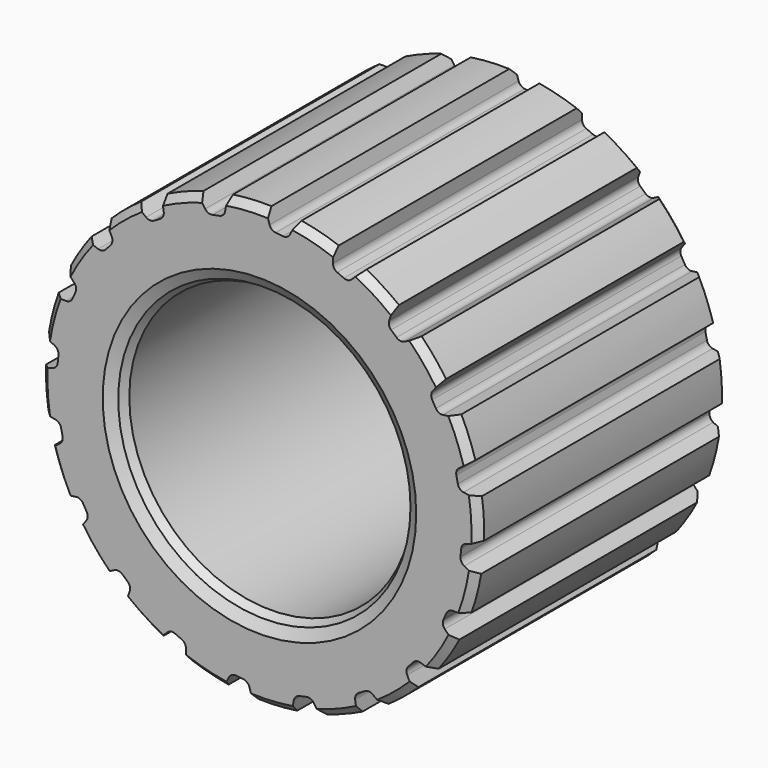
from build123d import *

# Parameters (mm, degrees)
F0_R            = 15.485
F0_R_2          = 10
F1_DEPTH        = 11
F2_SIZE2        = 0.5773502692
F2_SIZE         = 1
F3_SIZE2        = 0.5
F3_SIZE         = 0.5
F5_DEPTH        = 12.5
F5_COPIES_COUNT = 20
F6_SIZE2        = 0.5
F6_SIZE         = 0.5


# Not quite as in the source:
# - a pattern or mirror of a feature is missing from the dataset's text; its kind, count and spacing are read off the source's solid


with BuildPart() as f1:
    # F0 (on Front) → F1 (new body, symmetric)
    with BuildSketch(Plane.XZ):
        Circle(F0_R)
        Circle(F0_R_2, mode=Mode.SUBTRACT)
    extrude(amount=F1_DEPTH, both=True)

    # F2
    f2_edges = [f1.edges().sort_by_distance(p)[0] for p in [
        (-10, -11, 0),
        (-10, 11, 0),
    ]]
    f2_side = f1.faces().sort_by_distance((-10, 0, 0))[0]
    chamfer(f2_edges, length=F2_SIZE, length2=F2_SIZE2, reference=f2_side)

    # F3
    f3_edges = [f1.edges().sort_by_distance(p)[0] for p in [
        (-10.57735, -11, 0),
        (-10.57735, 11, 0),
    ]]
    chamfer(f3_edges, length=F3_SIZE, length2=F3_SIZE2)

    # F4 (on Front) → F5 (cut, symmetric)
    with BuildSketch(Plane.XZ):
        with BuildLine():
            Line((-2.4258394789, 14.4213544606), (-2.2677279827, 15.3180493143))
            ThreePointArc((-2.2677279827, 15.3180493143), (-3.319655777, 15.1249829925), (-4.3557481049, 14.8597672743))
            Line((-4.3557481049, 14.8597672743), (-3.8334908043, 14.1139065515))
            ThreePointArc((-3.8334908043, 14.1139065515), (-3.6071653955, 13.9354859857), (-3.3199589368, 13.9116209693))
            Line((-3.3199589368, 13.9116209693), (-2.81428751, 14.0191047491))
            ThreePointArc((-2.81428751, 14.0191047491), (-2.5585734552, 14.1608493642), (-2.4258394789, 14.4213544606))
        make_face()
    f5 = extrude(amount=F5_DEPTH, both=True, mode=Mode.SUBTRACT)

    # F5_copies: F5 ×20 about axis
    f5_copies_axis = Axis((0, 0, 0), (0, 1, 0))
    for i in range(1, F5_COPIES_COUNT):
        add(f5.rotate(f5_copies_axis, i * 360 / F5_COPIES_COUNT), mode=Mode.SUBTRACT)

    # F6
    f6_edges = [f1.edges().sort_by_distance(p)[0] for p in [
        (-15.458078, 11, -0.912717),
        (-15.458078, -11, -0.912717),
        (-0.912717, -11, 15.458078),
        (3.908764, -11, 14.983551),
        (8.347627, -11, 13.042329),
        (11.969366, -11, 9.824434),
        (14.419461, -11, 5.644854),
        (15.458078, -11, 0.912717),
        (14.983551, -11, -3.908764),
        (13.042329, -11, -8.347627),
        (9.824434, -11, -11.969366),
        (5.644854, -11, -14.419461),
        (0.912717, -11, -15.458078),
        (-3.908764, -11, -14.983551),
        (-8.347627, -11, -13.042329),
        (-11.969366, -11, -9.824434),
        (-14.419461, -11, -5.644854),
        (-14.983551, -11, 3.908764),
        (-13.042329, -11, 8.347627),
        (-9.824434, -11, 11.969366),
        (-5.644854, -11, 14.419461),
        (-0.912717, 11, 15.458078),
        (3.908764, 11, 14.983551),
        (8.347627, 11, 13.042329),
        (11.969366, 11, 9.824434),
        (14.419461, 11, 5.644854),
        (15.458078, 11, 0.912717),
        (14.983551, 11, -3.908764),
        (13.042329, 11, -8.347627),
        (9.824434, 11, -11.969366),
        (5.644854, 11, -14.419461),
        (0.912717, 11, -15.458078),
        (-3.908764, 11, -14.983551),
        (-8.347627, 11, -13.042329),
        (-11.969366, 11, -9.824434),
        (-14.419461, 11, -5.644854),
        (-14.983551, 11, 3.908764),
        (-13.042329, 11, 8.347627),
        (-9.824434, 11, 11.969366),
        (-5.644854, 11, 14.419461),
    ]]
    chamfer(f6_edges, length=F6_SIZE, length2=F6_SIZE2)


solid = f1.part
